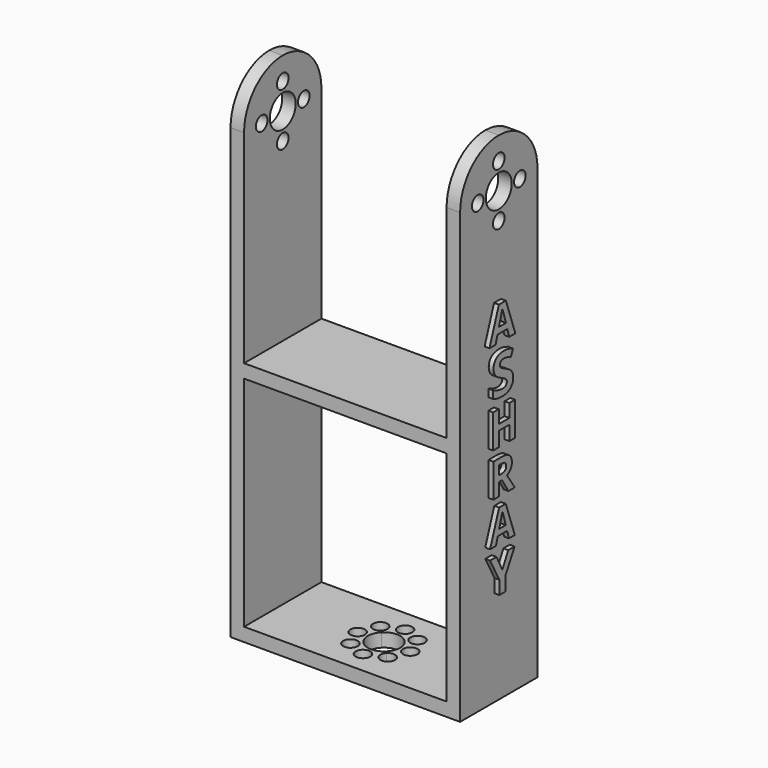
from build123d import *

# Parameters (mm, degrees)
F0_W            = 60.325
F0_H            = 25.4
F1_DEPTH        = 3.556
F2_W            = 3.556
F2_H            = 25.4
F3_DEPTH        = 127
F4_R            = 12.7
F5_R            = 12.69999
F6_R            = 4.2545
F6_R_2          = 1.905
F7_DEPTH        = 254
F10_TEXT_SIZE   = 11.7772717864
F10_TEXT_SIZE_2 = 14.1088147545
F10_TEXT_SIZE_3 = 12.0185889311
F10_TEXT_SIZE_4 = 12.2620689655
F10_TEXT_SIZE_5 = 12.9045134951
F11_DEPTH       = 1.27
F8_R            = 1.905
F13_DEPTH       = 25.4
F14_TEXT_SIZE   = 12.3472222222
F14_TEXT_SIZE_2 = 14.1088147545
F14_TEXT_SIZE_3 = 11.7772717864
F14_TEXT_SIZE_4 = 12.9045134951
F15_DEPTH       = 1.27
F9_W            = 25.4
F9_H            = 3.556
F16_DEPTH       = 53.34


# Not quite as in the source:
# - a fillet or chamfer is up to 0.001 mm smaller than in the source, because OpenCascade refuses the exact size
# - Text() gives the source's letters only with a copy of the font that has no kerning and outlines rounded to 1/6400 em; it was checked with that copy


with BuildPart() as f1:
    # F0 (on Top) → F1 (new body)
    with BuildSketch(Plane.XY):
        with Locations((3.8735, 0)):
            Rectangle(F0_W, F0_H)
    extrude(amount=F1_DEPTH)

    # F2 (on face) → F3 (join)
    with BuildSketch(Plane.XY.offset(3.556)):
        with Locations((-24.511, 0)):
            Rectangle(F2_W, F2_H)
        with Locations((32.258, 0)):
            Rectangle(F2_W, F2_H)
    extrude(amount=F3_DEPTH)

    # F4
    f4_edges = [f1.edges().sort_by_distance(p)[0] for p in [
        (32.258, 12.7, 130.556),
    ]]
    fillet(f4_edges, radius=F4_R)

    # F5 (radius 12.7 in the source; OpenCascade refuses exactly that, so slightly less here)
    f5_edges = [f1.edges().sort_by_distance(p)[0] for p in [
        (32.258, -12.7, 130.556),
        (-24.511, -12.7, 130.556),
        (-24.511, 12.7, 130.556),
    ]]
    fillet(f5_edges, radius=F5_R)

    # F6 (on face) → F7 (cut)
    with BuildSketch(Plane.YZ.offset(34.036)):
        with Locations((0, 117.6655)):
            Circle(F6_R)
        with Locations((0, 124.587)):
            Circle(F6_R_2)
        with Locations((-6.9215, 117.6655)):
            Circle(F6_R_2)
        with Locations((0, 110.744)):
            Circle(F6_R_2)
        with Locations((6.9215, 117.6655)):
            Circle(F6_R_2)
    extrude(amount=-F7_DEPTH, mode=Mode.SUBTRACT)

    # F10 (on face) → F11 (join)
    with BuildSketch(Plane(origin=(-26.289, 0, 0), x_dir=(0, -1, 0), z_dir=(-1, 0, 0))):
        with Locations((-4.445, 83.9763643138)):
            Text('A', F10_TEXT_SIZE, font='Open Sans', font_style=FontStyle.BOLD, text_align=(TextAlign.LEFT, TextAlign.BOTTOM))
        with Locations((-4.064, 71.2780176905)):
            Text('S', F10_TEXT_SIZE_2, font='Open Sans', font_style=FontStyle.BOLD, text_align=(TextAlign.LEFT, TextAlign.BOTTOM))
        with Locations((-4.445, 60.0846336601)):
            Text('H', F10_TEXT_SIZE_3, font='Open Sans', font_style=FontStyle.BOLD, text_align=(TextAlign.LEFT, TextAlign.BOTTOM))
        with Locations((-4.445, 48.7159440049)):
            Text('R', F10_TEXT_SIZE_4, font='Open Sans', font_style=FontStyle.BOLD, text_align=(TextAlign.LEFT, TextAlign.BOTTOM))
        with Locations((-4.445, 37.6963083188)):
            Text('A', F10_TEXT_SIZE, font='Open Sans', font_style=FontStyle.BOLD, text_align=(TextAlign.LEFT, TextAlign.BOTTOM))
        with Locations((-4.445, 25.8650586023)):
            Text('Y', F10_TEXT_SIZE_5, font='Open Sans', font_style=FontStyle.BOLD, text_align=(TextAlign.LEFT, TextAlign.BOTTOM))
    extrude(amount=F11_DEPTH)

    # F8 (on face) → F13 (cut)
    with BuildSketch(Plane.XY.offset(3.556)):
        with BuildLine():
            ThreePointArc((10.672739586, 4.894239586), (8.0387276473, 6.6542300954), (7.4207011678, 3.5472011678))
            ThreePointArc((7.4207011678, 3.5472011678), (9.4967515246, 3.1342490765), (10.672739586, 4.894239586))
        make_face()
        with Locations((10.795, 0)):
            Circle(F8_R)
        with BuildLine():
            ThreePointArc((10.672739586, -4.894239586), (9.4967515246, -3.1342490765), (7.4207011678, -3.5472011678))
            ThreePointArc((7.4207011678, -3.5472011678), (8.0387276473, -6.6542300954), (10.672739586, -4.894239586))
        make_face()
        with Locations((3.8735, -6.9215)):
            Circle(F8_R)
        with BuildLine():
            ThreePointArc((0.884260414, -4.894239586), (0.7392509235, -4.1652276473), (0.3262988322, -3.5472011678))
            ThreePointArc((0.3262988322, -3.5472011678), (-2.7807300954, -5.6232515246), (0.884260414, -4.894239586))
        make_face()
        with Locations((-3.048, 0)):
            Circle(F8_R)
        with BuildLine():
            ThreePointArc((0.884260414, 4.894239586), (-2.7807300954, 5.6232515246), (0.3262988322, 3.5472011678))
            ThreePointArc((0.3262988322, 3.5472011678), (0.7392509235, 4.1652276473), (0.884260414, 4.894239586))
        make_face()
        with Locations((3.8735, 6.9215)):
            Circle(F8_R)
        with BuildLine():
            Line((3.8735, 0), (6.8818858006, 3.0083858006))
            ThreePointArc((6.8818858006, 3.0083858006), (3.8735, 4.2545), (0.8651141994, 3.0083858006))
            Line((0.8651141994, 3.0083858006), (3.8735, 0))
        make_face()
        with BuildLine():
            Line((3.8735, 0), (0.8651141994, 3.0083858006))
            ThreePointArc((0.8651141994, 3.0083858006), (-0.381, 0), (0.8651141994, -3.0083858006))
            Line((0.8651141994, -3.0083858006), (3.8735, 0))
        make_face()
        with BuildLine():
            ThreePointArc((0.8651141994, -3.0083858006), (3.8735, -4.2545), (6.8818858006, -3.0083858006))
            Line((6.8818858006, -3.0083858006), (3.8735, 0))
            Line((3.8735, 0), (0.8651141994, -3.0083858006))
        make_face()
        with BuildLine():
            ThreePointArc((6.8818858006, -3.0083858006), (7.8041454711, -1.628126663), (8.128, 0))
            ThreePointArc((8.128, 0), (7.8041454711, 1.628126663), (6.8818858006, 3.0083858006))
            Line((6.8818858006, 3.0083858006), (3.8735, 0))
            Line((3.8735, 0), (6.8818858006, -3.0083858006))
        make_face()
    extrude(amount=-F13_DEPTH, mode=Mode.SUBTRACT)

    # F14 (on face) → F15 (join)
    with BuildSketch(Plane.YZ.offset(34.036)):
        with Locations((-4.6601117622, 83.566)):
            Text('A', F14_TEXT_SIZE, font='Open Sans', font_style=FontStyle.BOLD, text_align=(TextAlign.LEFT, TextAlign.BOTTOM))
        with Locations((-4.064, 70.8676533767)):
            Text('S', F14_TEXT_SIZE_2, font='Open Sans', font_style=FontStyle.BOLD, text_align=(TextAlign.LEFT, TextAlign.BOTTOM))
        with Locations((-4.5665429688, 59.4376533767)):
            Text('H', F14_TEXT_SIZE, font='Open Sans', font_style=FontStyle.BOLD, text_align=(TextAlign.LEFT, TextAlign.BOTTOM))
        with Locations((-4.4758680556, 48.0076533767)):
            Text('R', F14_TEXT_SIZE, font='Open Sans', font_style=FontStyle.BOLD, text_align=(TextAlign.LEFT, TextAlign.BOTTOM))
        with Locations((-4.445, 36.9880176905)):
            Text('A', F14_TEXT_SIZE_3, font='Open Sans', font_style=FontStyle.BOLD, text_align=(TextAlign.LEFT, TextAlign.BOTTOM))
        with Locations((-4.445, 25.156767974)):
            Text('Y', F14_TEXT_SIZE_4, font='Open Sans', font_style=FontStyle.BOLD, text_align=(TextAlign.LEFT, TextAlign.BOTTOM))
    extrude(amount=F15_DEPTH)

    # F9 (on face) → F16 (join)
    with BuildSketch(Plane(origin=(30.48, 0, 0), x_dir=(0, -1, 0), z_dir=(-1, 0, 0))):
        with Locations((0, 62.738)):
            Rectangle(F9_W, F9_H)
    extrude(amount=F16_DEPTH)


solid = f1.part
